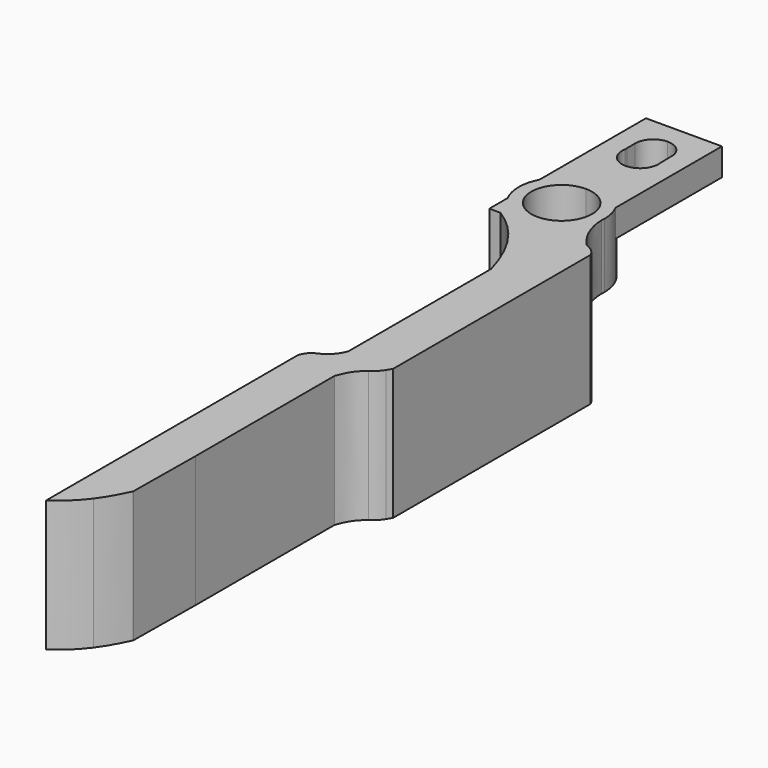
from build123d import *

# Parameters (mm, degrees)
F1_DEPTH = 5.9
F2_DEPTH = 2.5
F3_DEPTH = 5.9
F4_DEPTH = 12
F5_DEPTH = 12


with BuildPart() as f1:
    # F0 (on Top) → F1 (new body)
    with BuildSketch(Plane.XY):
        with BuildLine():
            Line((3.475, 1.15), (3.475, 0))
            ThreePointArc((3.475, 0), (4.7730375063, 0.2208504846), (5.925, 0.8585484677))
            ThreePointArc((5.925, 0.8585484677), (6.5018486959, 1.426237912), (6.95, 2.1001712409))
            Line((6.95, 2.1001712409), (6.95, 5.7498287591))
            ThreePointArc((6.95, 5.7498287591), (5.5051689733, 7.2841723593), (3.475, 7.85))
            Line((3.475, 7.85), (3.475, 6.8908035755))
            Line((3.475, 6.8908035755), (3.475, 6.7))
            ThreePointArc((3.475, 6.7), (5.4372213178, 5.8872213178), (6.25, 3.925))
            ThreePointArc((6.25, 3.925), (5.4372213178, 1.9627786822), (3.475, 1.15))
        make_face()
        with BuildLine():
            Line((6.95, 5.7498287591), (6.95, 2.1001712409))
            ThreePointArc((6.95, 2.1001712409), (7.2391359007, 2.8128372775), (7.3837493972, 3.5682043308))
            ThreePointArc((7.3837493972, 3.5682043308), (7.3959352446, 3.7464172239), (7.4, 3.925))
            ThreePointArc((7.4, 3.925), (7.2858398025, 4.8647473065), (6.95, 5.7498287591))
        make_face()
        with BuildLine():
            Line((0, 5.7498287591), (0, 2.1001712409))
            ThreePointArc((0, 2.1001712409), (0.4481513041, 1.426237912), (1.025, 0.8585484677))
            ThreePointArc((1.025, 0.8585484677), (2.1769624937, 0.2208504846), (3.475, 0))
            Line((3.475, 0), (3.475, 1.15))
            ThreePointArc((3.475, 1.15), (0.7, 3.925), (3.475, 6.7))
            Line((3.475, 6.7), (3.475, 6.8908035755))
            Line((3.475, 6.8908035755), (3.475, 7.85))
            ThreePointArc((3.475, 7.85), (1.4448310267, 7.2841723593), (0, 5.7498287591))
        make_face()
        with BuildLine():
            ThreePointArc((0, 5.7498287591), (-0.45, 3.925), (0, 2.1001712409))
            Line((0, 2.1001712409), (0, 5.7498287591))
        make_face()
        with BuildLine():
            ThreePointArc((6.95, 2.1001712409), (6.5018486959, 1.426237912), (5.925, 0.8585484677))
            Line((5.925, 0.8585484677), (5.925, 0))
            Line((5.925, 0), (6.95, 0))
            Line((6.95, 0), (6.95, 0.75))
            Line((6.95, 0.75), (6.95, 1.44))
            Line((6.95, 1.44), (6.95, 1.5))
            Line((6.95, 1.5), (6.95, 2.1001712409))
        make_face()
        with BuildLine():
            Line((0, 2.1001712409), (0, 0))
            Line((0, 0), (1.025, 0))
            Line((1.025, 0), (1.025, 0.8585484677))
            ThreePointArc((1.025, 0.8585484677), (0.4481513041, 1.426237912), (0, 2.1001712409))
        make_face()
        with BuildLine():
            Line((1.025, 0.8585484677), (1.025, 0))
            Line((1.025, 0), (3.475, 0))
            ThreePointArc((3.475, 0), (2.1769624937, 0.2208504846), (1.025, 0.8585484677))
        make_face()
        with BuildLine():
            ThreePointArc((5.925, 0.8585484677), (4.7730375063, 0.2208504846), (3.475, 0))
            Line((3.475, 0), (4.7, 0))
            Line((4.7, 0), (5.925, 0))
            Line((5.925, 0), (5.925, 0.8585484677))
        make_face()
        with BuildLine():
            Line((5.925, 0), (4.7, 0))
            add(Edge.make_bspline(
                [(4.7, 0), (5.2537494339, -0.3164176305), (5.6369397789, -0.7196032093), (5.925, -1.225)],
                knots=[0, 0, 0, 0, 1.7324116139, 1.7324116139, 1.7324116139, 1.7324116139], degree=3))
            Line((5.925, -1.225), (5.925, -0.079424061))
            Line((5.925, -0.079424061), (5.925, 0))
        make_face()
        with BuildLine():
            Line((6.95, 0.75), (6.95, 0))
            Line((6.95, 0), (7.9496195498, -0.0275818011))
            add(Edge.make_bspline(
                [(7.9496195498, -0.0275818011), (7.5186002068, 0.1973926119), (7.1600275114, 0.4521599913), (6.95, 0.75)],
                knots=[0, 0, 0, 0, 1.2664409586, 1.2664409586, 1.2664409586, 1.2664409586], degree=3))
        make_face()
    extrude(amount=-F1_DEPTH)

    # F0 (on Top) → F2 (join)
    with BuildSketch(Plane.XY):
        with BuildLine():
            Line((0, 7.85), (0, 5.7498287591))
            ThreePointArc((0, 5.7498287591), (1.4448310267, 7.2841723593), (3.475, 7.85))
            ThreePointArc((3.475, 7.85), (5.5051689733, 7.2841723593), (6.95, 5.7498287591))
            Line((6.95, 5.7498287591), (6.95, 17.9))
            Line((6.95, 17.9), (3.475, 17.9))
            Line((3.475, 17.9), (0, 17.9))
            Line((0, 17.9), (0, 7.85))
        make_face()
        with BuildLine():
            ThreePointArc((1.8276640256, 14.3833613398), (2.3042302705, 15.55900427), (3.475, 16.0474200003))
            ThreePointArc((3.475, 16.0474200003), (4.5253988967, 15.6691157612), (5.0933824344, 14.7079463483))
            Line((5.0933824344, 14.7079463483), (5.1024433757, 14.1442252627))
            Line((5.1024433757, 14.1442252627), (5.113982201, 13.4263440945))
            ThreePointArc((5.113982201, 13.4263440945), (5.1141409801, 13.4131724726), (5.1141939076, 13.4))
            ThreePointArc((5.1141939076, 13.4), (5.1117771913, 13.3110219533), (5.1045341684, 13.222306273))
            ThreePointArc((5.1045341684, 13.222306273), (5.1281919004, 13.0619243035), (5.1361029286, 12.9))
            ThreePointArc((5.1361029286, 12.9), (5.0161594238, 12.2802495905), (4.673650466, 11.75))
            ThreePointArc((4.673650466, 11.75), (3.475, 11.2388970714), (2.276349534, 11.75))
            ThreePointArc((2.276349534, 11.75), (1.8807671055, 12.4334333727), (1.8454658316, 13.222306273))
            ThreePointArc((1.8454658316, 13.222306273), (1.8368359194, 13.3419042896), (1.8369719791, 13.4618131819))
            Line((1.8369719791, 13.4618131819), (1.8276640256, 14.3833613398))
        make_face(mode=Mode.SUBTRACT)
    extrude(amount=-F2_DEPTH)

    # F0 (on Top) → F3 (join)
    with BuildSketch(Plane.XY):
        with BuildLine():
            Line((6.95, 5.7498287591), (6.95, 2.1001712409))
            ThreePointArc((6.95, 2.1001712409), (7.2391359007, 2.8128372775), (7.3837493972, 3.5682043308))
            ThreePointArc((7.3837493972, 3.5682043308), (7.3959352446, 3.7464172239), (7.4, 3.925))
            ThreePointArc((7.4, 3.925), (7.2858398025, 4.8647473065), (6.95, 5.7498287591))
        make_face()
        with BuildLine():
            Line((6.95, 0.75), (6.95, 0))
            Line((6.95, 0), (7.9496195498, -0.0275818011))
            add(Edge.make_bspline(
                [(7.9496195498, -0.0275818011), (7.5186002068, 0.1973926119), (7.1600275114, 0.4521599913), (6.95, 0.75)],
                knots=[0, 0, 0, 0, 1.2664409586, 1.2664409586, 1.2664409586, 1.2664409586], degree=3))
        make_face()
        with BuildLine():
            ThreePointArc((7.3837493972, 3.5682043308), (7.2391359007, 2.8128372775), (6.95, 2.1001712409))
            Line((6.95, 2.1001712409), (6.95, 1.5))
            Line((6.95, 1.5), (6.95, 1.44))
            Line((6.95, 1.44), (6.95, 0.75))
            add(Edge.make_bspline(
                [(7.9496195498, -0.0275818011), (7.5186002068, 0.1973926119), (7.1600275114, 0.4521599913), (6.95, 0.75)],
                knots=[0, 0, 0, 0, 1.2664409586, 1.2664409586, 1.2664409586, 1.2664409586], degree=3))
            Line((7.9496195498, -0.0275818011), (8.9492390995, -0.0551636022))
            add(Edge.make_bspline(
                [(8.9492390995, -0.0551636022), (7.8965900466, 1.0567778954), (7.4345106259, 2.2768541239), (7.3837493972, 3.5682043308)],
                knots=[0, 0, 0, 0, 3.9470942713, 3.9470942713, 3.9470942713, 3.9470942713], degree=3))
        make_face()
        with BuildLine():
            Line((3.475, 0), (1.025, 0))
            add(Edge.make_bspline(
                [(1.025, 0), (1.9679788021, -0.5904915447), (2.7813095381, -1.3164345806), (3.475, -2.169177953)],
                knots=[0, 0, 0, 0, 3.3501258039, 3.3501258039, 3.3501258039, 3.3501258039], degree=3))
            Line((3.475, -2.169177953), (3.475, -1.225))
            Line((3.475, -1.225), (3.475, 0))
        make_face()
        with BuildLine():
            Line((4.7, 0), (3.475, 0))
            Line((3.475, 0), (3.475, -1.225))
            Line((3.475, -1.225), (3.475, -2.169177953))
            add(Edge.make_bspline(
                [(3.475, -2.169177953), (4.583621136, -3.5319894349), (5.386671183, -5.2186593933), (5.925, -7.1938754991)],
                knots=[3.3501258039, 3.3501258039, 3.3501258039, 3.3501258039, 8.7041280262, 8.7041280262, 8.7041280262, 8.7041280262], degree=3))
            Line((5.925, -7.1938754991), (5.925, -1.225))
            add(Edge.make_bspline(
                [(4.7, 0), (5.2537494339, -0.3164176305), (5.6369397789, -0.7196032093), (5.925, -1.225)],
                knots=[0, 0, 0, 0, 1.7324116139, 1.7324116139, 1.7324116139, 1.7324116139], degree=3))
        make_face()
    extrude(amount=-F3_DEPTH)

    # F0 (on Top) → F4 (join)
    with BuildSketch(Plane.XY):
        with BuildLine():
            Line((5.925, -1.225), (5.925, -7.1938754991))
            Line((5.925, -7.1938754991), (5.925, -21.3844068348))
            Line((5.925, -21.3844068348), (5.925, -22.55))
            Line((5.925, -22.55), (5.925, -22.9875))
            Line((5.925, -22.9875), (5.925, -23.5205553472))
            Line((5.925, -23.5205553472), (5.925, -25))
            Line((5.925, -25), (7.525, -25))
            Line((7.525, -25), (8.9492390995, -25))
            Line((8.9492390995, -25), (8.9492390995, -0.9913714603))
            add(Edge.make_bspline(
                [(7.9496195498, -0.0275818011), (8.4295123816, -0.2455351059), (8.7658986449, -0.6068330258), (8.9492390995, -0.9913714603)],
                knots=[0, 0, 0, 0, 1.3885711186, 1.3885711186, 1.3885711186, 1.3885711186], degree=3))
            Line((7.9496195498, -0.0275818011), (6.95, 0))
            Line((6.95, 0), (5.925, 0))
            Line((5.925, 0), (5.925, -0.079424061))
            Line((5.925, -0.079424061), (5.925, -1.225))
        make_face()
        with BuildLine():
            add(Edge.make_bspline(
                [(4.7, -25), (4.0586842224, -25.2618398517), (3.6450892221, -25.6055109203), (3.475, -26.225)],
                knots=[0, 0, 0, 0, 1.7324116139, 1.7324116139, 1.7324116139, 1.7324116139], degree=3))
            Line((3.475, -26.225), (3.475, -48.775))
            Line((3.475, -48.775), (3.475, -50))
            Line((3.475, -50), (5.925, -50))
            Line((5.925, -50), (5.925, -47.55))
            Line((5.925, -47.55), (5.925, -43))
            Line((5.925, -43), (5.925, -28.903))
            Line((5.925, -28.903), (5.925, -26.9515))
            Line((5.925, -26.9515), (5.925, -25))
            Line((5.925, -25), (4.7, -25))
        make_face()
        with BuildLine():
            add(Edge.make_bspline(
                [(4.7, -25), (5.3314492106, -24.6048551053), (5.6424522772, -24.1878218949), (5.925, -23.5205553472)],
                knots=[0, 0, 0, 0, 1.9207762703, 1.9207762703, 1.9207762703, 1.9207762703], degree=3))
            Line((4.7, -25), (5.925, -25))
            Line((5.925, -25), (5.925, -23.5205553472))
        make_face()
        with BuildLine():
            Line((8.9492390995, -0.0551636022), (7.9496195498, -0.0275818011))
            add(Edge.make_bspline(
                [(7.9496195498, -0.0275818011), (8.4295123816, -0.2455351059), (8.7658986449, -0.6068330258), (8.9492390995, -0.9913714603)],
                knots=[0, 0, 0, 0, 1.3885711186, 1.3885711186, 1.3885711186, 1.3885711186], degree=3))
            Line((8.9492390995, -0.9913714603), (8.9492390995, -0.0551636022))
        make_face()
        with BuildLine():
            add(Edge.make_bspline(
                [(8.9492390995, -0.0551636022), (9.326442021, -0.1917248564), (9.6147849957, -0.3848434336), (9.8284865708, -0.6283950562)],
                knots=[0, 0, 0, 0, 1.0008605929, 1.0008605929, 1.0008605929, 1.0008605929], degree=3))
            Line((8.9492390995, -0.0551636022), (8.9492390995, -0.9913714603))
            Line((8.9492390995, -0.9913714603), (8.9492390995, -25))
            add(Edge.make_bspline(
                [(8.9492390995, -25), (9.331126801, -24.7616745123), (9.6040893739, -24.433150219), (9.8284865708, -24.0874149632)],
                knots=[0, 0, 0, 0, 1.2440499597, 1.2440499597, 1.2440499597, 1.2440499597], degree=3))
            Line((9.8284865708, -24.0874149632), (9.8284865708, -0.6283950562))
        make_face()
        Polygon((7.525, -25), (5.925, -25), (5.925, -26.9515), (5.925, -28.903), (5.925, -43), (7.525, -43), (7.525, -27.1006729454), align=None)
        with BuildLine():
            add(Edge.make_bspline(
                [(9.8284865708, -0.6283950562), (9.942237153, -0.7580344322), (10.0348396241, -0.9019629784), (10.1084383205, -1.0592570761)],
                knots=[1.0008605929, 1.0008605929, 1.0008605929, 1.0008605929, 1.533605731, 1.533605731, 1.533605731, 1.533605731], degree=3))
            Line((9.8284865708, -0.6283950562), (9.8284865708, -24.0874149632))
            add(Edge.make_bspline(
                [(9.8284865708, -24.0874149632), (9.9298603822, -23.9312253982), (10.0213226008, -23.7715232886), (10.1084383205, -23.6150380224)],
                knots=[1.2440499597, 1.2440499597, 1.2440499597, 1.2440499597, 1.8060627102, 1.8060627102, 1.8060627102, 1.8060627102], degree=3))
            Line((10.1084383205, -23.6150380224), (10.1084383205, -1.0592570761))
        make_face()
        with BuildLine():
            Line((5.925, -50), (3.475, -50))
            Line((3.475, -50), (3.475, -55))
            add(Edge.make_bspline(
                [(3.475, -55), (4.512583722, -54.3078648135), (5.2908616095, -53.5264365704), (5.925, -52.6706067544)],
                knots=[0, 0, 0, 0, 3.2551675464, 3.2551675464, 3.2551675464, 3.2551675464], degree=3))
            Line((5.925, -52.6706067544), (5.925, -52.0125))
            Line((5.925, -52.0125), (5.925, -50))
        make_face()
        with BuildLine():
            Line((8.9492390995, -25), (7.525, -25))
            Line((7.525, -25), (7.525, -27.1006729454))
            add(Edge.make_bspline(
                [(8.9492390995, -25), (8.2447035238, -25.5232192576), (7.9111177474, -26.03264153), (7.525, -27.1006729454)],
                knots=[0, 0, 0, 0, 2.5379684466, 2.5379684466, 2.5379684466, 2.5379684466], degree=3))
        make_face()
        with BuildLine():
            Line((7.4536274492, -50.0155514561), (5.925, -50))
            Line((5.925, -50), (5.925, -52.0125))
            Line((5.925, -52.0125), (5.925, -52.6706067544))
            add(Edge.make_bspline(
                [(5.925, -52.6706067544), (6.5332867434, -51.8496661845), (7.0089465882, -50.9602665865), (7.4536274492, -50.0155514561)],
                knots=[3.2551675464, 3.2551675464, 3.2551675464, 3.2551675464, 6.3776330772, 6.3776330772, 6.3776330772, 6.3776330772], degree=3))
        make_face()
        Polygon((5.925, -47.55), (5.925, -50), (7.4537856616, -50), (7.525, -43), (5.925, -43), align=None)
    extrude(amount=-F4_DEPTH)

    # F0 (on Top) → F5 (join)
    with BuildSketch(Plane.XY):
        Polygon((7.4537856616, -50), (5.925, -50), (7.4536274492, -50.0155514561), align=None)
    extrude(amount=-F5_DEPTH)


solid = f1.part
